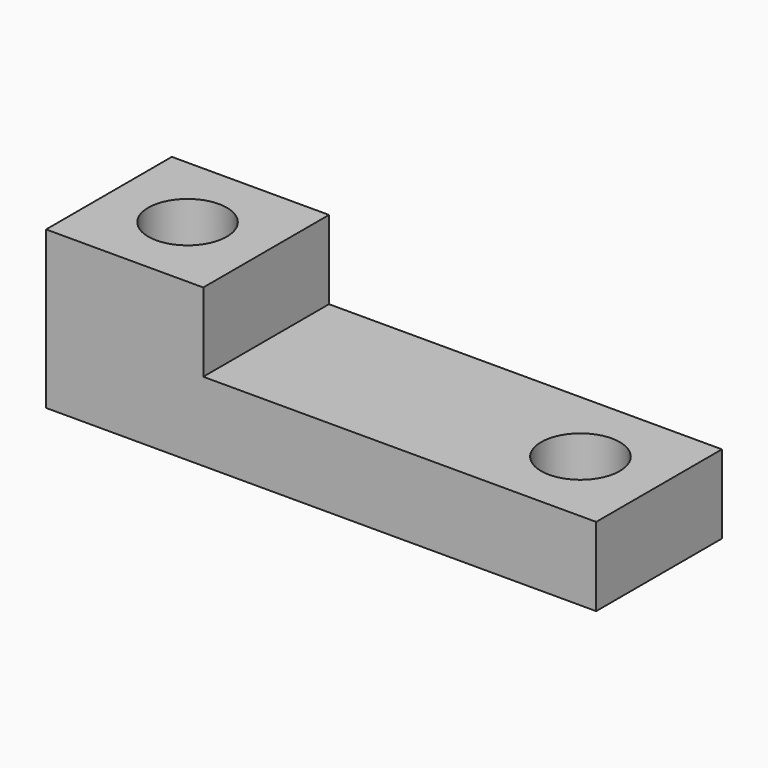
from build123d import *

# Parameters (mm, degrees)
F1_DEPTH = 12.7
F3_D     = 12.7


# Not quite as in the source:
# - a length typed as a fraction of an inch, garbled in the dataset ("3 / 203.2 mm" for 3/8 in), is restored


with BuildPart() as f1:
    # F0 (on Front) → F1 (new body, symmetric)
    with BuildSketch(Plane.XZ):
        Polygon((0, -12.7), (0, 0), (-63.5, 0), (-63.5, 12.7), (-88.9, 12.7), (-88.9, -12.7), align=None)
    extrude(amount=F1_DEPTH, both=True)

    # F3 (through all)
    with Locations(Plane(origin=(0, 0, -12.7), x_dir=(1, 0, 0), z_dir=(0, 0, -1))):
        with Locations((-76.2, 0), (-12.7, 0)):
            Hole(F3_D / 2)


solid = f1.part
